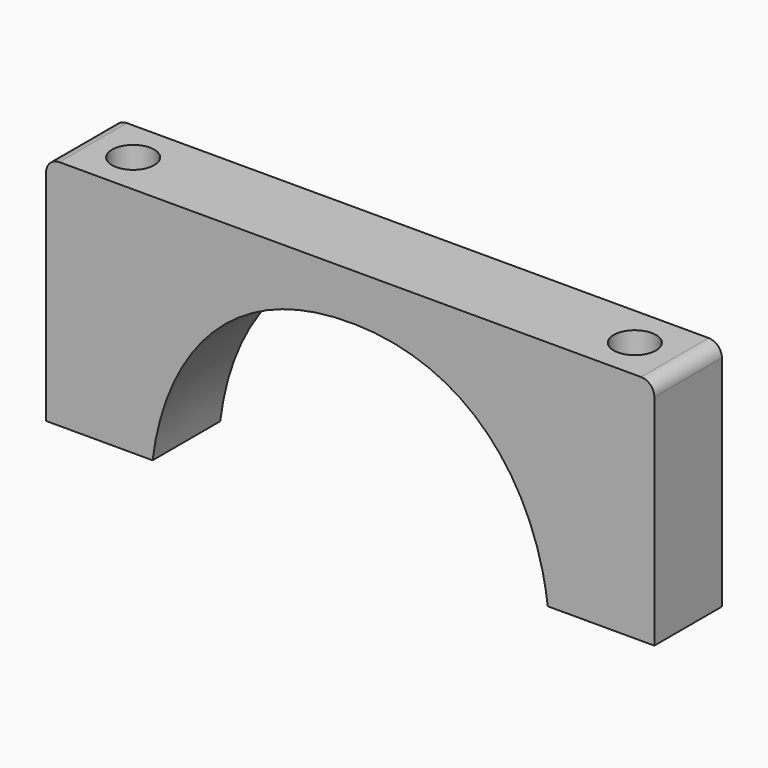
from build123d import *

# Parameters (mm, degrees)
F1_DEPTH = 12.7
F2_R     = 3.175
F3_DEPTH = 34.9
F4_R     = 3.175
F5_DEPTH = 34.9
F6_R     = 2


with BuildPart() as f1:
    # F0 (on Front) → F1 (new body)
    with BuildSketch(Plane.XZ):
        with BuildLine():
            Line((-5.8658062685, 5), (0.3025391327, 5))
            add(Edge.make_bspline(
                [(0.3025391327, 5), (2.0272433596, 19.1776482129), (11.2100582813, 32.9), (30, 32.9)],
                knots=[4.6857722032, 4.6857722032, 4.6857722032, 4.6857722032, 44.5242630484, 44.5242630484, 44.5242630484, 44.5242630484], degree=3))
            add(Edge.make_bspline(
                [(59.6974608673, 5), (57.9727566404, 19.1776482129), (48.7899417187, 32.9), (30, 32.9)],
                knots=[4.6857722032, 4.6857722032, 4.6857722032, 4.6857722032, 44.5242630484, 44.5242630484, 44.5242630484, 44.5242630484], degree=3))
            Line((59.6974608673, 5), (65.8658062685, 5))
            add(Edge.make_bspline(
                [(65.8658062685, 5), (65.8175694138, 5.6045543906), (65.5206979037, 8.5111158621), (64.3376946497, 13.6666771768), (61.7778690019, 20.2490905933), (57.9831497379, 26.3746466103), (52.8726260404, 31.7533398634), (46.3887061881, 35.9435716124), (39.581089223, 38.4154216198), (34.9653521704, 38.8398717945), (33.0331003636, 38.9)],
                knots=[5.0019704128, 5.0019704128, 5.0019704128, 5.0019704128, 6.8206255364, 13.7629955356, 20.7886344542, 27.9249237942, 35.2442046754, 42.8555124684, 50.901123614, 56.6904025365, 56.6904025365, 56.6904025365, 56.6904025365], degree=3))
            Line((33.0331003636, 38.9), (30, 38.9))
            Line((30, 38.9), (26.9668996364, 38.9))
            add(Edge.make_bspline(
                [(-5.8658062685, 5), (-5.8175694138, 5.6045543906), (-5.5206979037, 8.5111158621), (-4.3376946497, 13.6666771768), (-1.7778690019, 20.2490905933), (2.0168502621, 26.3746466103), (7.1273739596, 31.7533398634), (13.6112938119, 35.9435716124), (20.418910777, 38.4154216198), (25.0346478296, 38.8398717945), (26.9668996364, 38.9)],
                knots=[5.0019704128, 5.0019704128, 5.0019704128, 5.0019704128, 6.8206255364, 13.7629955356, 20.7886344542, 27.9249237942, 35.2442046754, 42.8555124684, 50.901123614, 56.6904025365, 56.6904025365, 56.6904025365, 56.6904025365], degree=3))
        make_face()
        with BuildLine():
            Line((-15.7074608673, 5), (-5.8658062685, 5))
            add(Edge.make_bspline(
                [(-5.8658062685, 5), (-5.8175694138, 5.6045543906), (-5.5206979037, 8.5111158621), (-4.3376946497, 13.6666771768), (-1.7778690019, 20.2490905933), (2.0168502621, 26.3746466103), (7.1273739596, 31.7533398634), (13.6112938119, 35.9435716124), (20.418910777, 38.4154216198), (25.0346478296, 38.8398717945), (26.9668996364, 38.9)],
                knots=[5.0019704128, 5.0019704128, 5.0019704128, 5.0019704128, 6.8206255364, 13.7629955356, 20.7886344542, 27.9249237942, 35.2442046754, 42.8555124684, 50.901123614, 56.6904025365, 56.6904025365, 56.6904025365, 56.6904025365], degree=3))
            Line((26.9668996364, 38.9), (-15.7074608673, 38.9))
            Line((-15.7074608673, 38.9), (-15.7074608673, 5))
        make_face()
        with BuildLine():
            add(Edge.make_bspline(
                [(65.8658062685, 5), (65.8175694138, 5.6045543906), (65.5206979037, 8.5111158621), (64.3376946497, 13.6666771768), (61.7778690019, 20.2490905933), (57.9831497379, 26.3746466103), (52.8726260404, 31.7533398634), (46.3887061881, 35.9435716124), (39.581089223, 38.4154216198), (34.9653521704, 38.8398717945), (33.0331003636, 38.9)],
                knots=[5.0019704128, 5.0019704128, 5.0019704128, 5.0019704128, 6.8206255364, 13.7629955356, 20.7886344542, 27.9249237942, 35.2442046754, 42.8555124684, 50.901123614, 56.6904025365, 56.6904025365, 56.6904025365, 56.6904025365], degree=3))
            Line((65.8658062685, 5), (75.7074608673, 5))
            Line((75.7074608673, 5), (75.7074608673, 38.9))
            Line((75.7074608673, 38.9), (33.0331003636, 38.9))
        make_face()
        with BuildLine():
            Line((-15.7074608673, 38.9), (26.9668996364, 38.9))
            add(Edge.make_bspline(
                [(26.9668996364, 38.9), (27.9792387785, 38.9315021757), (28.9917902537, 38.9307560105), (30, 38.9)],
                knots=[56.6904025365, 56.6904025365, 56.6904025365, 56.6904025365, 59.7235029001, 59.7235029001, 59.7235029001, 59.7235029001], degree=3))
            add(Edge.make_bspline(
                [(33.0331003636, 38.9), (32.0207612215, 38.9315021757), (31.0082097463, 38.9307560105), (30, 38.9)],
                knots=[56.6904025365, 56.6904025365, 56.6904025365, 56.6904025365, 59.7235029001, 59.7235029001, 59.7235029001, 59.7235029001], degree=3))
            Line((33.0331003636, 38.9), (75.7074608673, 38.9))
            Line((75.7074608673, 38.9), (75.7074608673, 39.9))
            Line((75.7074608673, 39.9), (-15.7074608673, 39.9))
            Line((-15.7074608673, 39.9), (-15.7074608673, 38.9))
        make_face()
        with BuildLine():
            add(Edge.make_bspline(
                [(26.9668996364, 38.9), (27.9792387785, 38.9315021757), (28.9917902537, 38.9307560105), (30, 38.9)],
                knots=[56.6904025365, 56.6904025365, 56.6904025365, 56.6904025365, 59.7235029001, 59.7235029001, 59.7235029001, 59.7235029001], degree=3))
            Line((26.9668996364, 38.9), (30, 38.9))
        make_face()
        with BuildLine():
            Line((30, 38.9), (33.0331003636, 38.9))
            add(Edge.make_bspline(
                [(33.0331003636, 38.9), (32.0207612215, 38.9315021757), (31.0082097463, 38.9307560105), (30, 38.9)],
                knots=[56.6904025365, 56.6904025365, 56.6904025365, 56.6904025365, 59.7235029001, 59.7235029001, 59.7235029001, 59.7235029001], degree=3))
        make_face()
    extrude(amount=F1_DEPTH)

    # F2 (on face) → F3 (cut, through all)
    with BuildSketch(Plane(origin=(0, 0, 5), x_dir=(1, 0, 0), z_dir=(0, 0, -1))):
        with Locations((-7.6974608673, 6.35)):
            Circle(F2_R)
    extrude(amount=-F3_DEPTH, mode=Mode.SUBTRACT)

    # F4 (on face) → F5 (cut, through all)
    with BuildSketch(Plane(origin=(0, 0, 5), x_dir=(1, 0, 0), z_dir=(0, 0, -1))):
        with Locations((67.6974608673, 6.35)):
            Circle(F4_R)
    extrude(amount=-F5_DEPTH, mode=Mode.SUBTRACT)

    # F6
    f6_edges = [f1.edges().sort_by_distance(p)[0] for p in [
        (-15.707461, -6.35, 39.9),
        (75.707461, -6.35, 39.9),
    ]]
    fillet(f6_edges, radius=F6_R)


solid = f1.part
